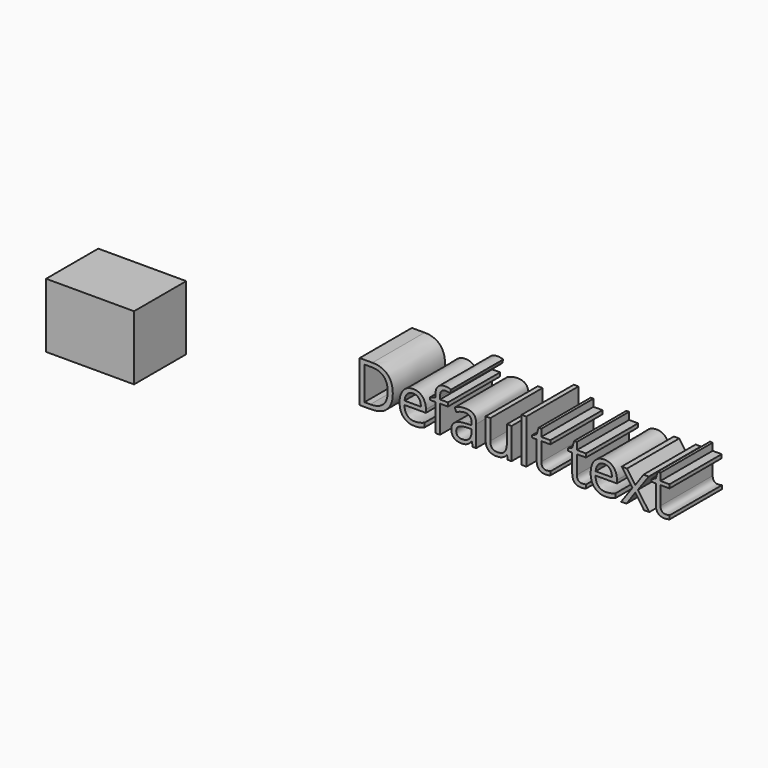
from build123d import *

# Parameters (mm, degrees)
F0_W         = 34.244004637
F0_H         = 25.0763148069
F1_DEPTH     = 25.4
F2_TEXT_SIZE = 22.6190003256
F3_DEPTH     = 25.4


# Not quite as in the source:
# - Text() gives the source's letters only with a copy of the font that has no kerning and outlines rounded to 1/6400 em; it was checked with that copy


with BuildPart() as f1:
    # F0 (on Front) → F1 (new body)
    with BuildSketch(Plane.XZ):
        with Locations((-53.9956521243, 29.0821269155)):
            Rectangle(F0_W, F0_H)
    extrude(amount=F1_DEPTH)


with BuildPart() as f3:
    # F2 (on face) → F3 (new body)
    with BuildSketch(Plane.XZ.offset(25.4)):
        with Locations((69.0735951066, 54.9350082874)):
            Text('Default text', F2_TEXT_SIZE, font='Open Sans', text_align=(TextAlign.LEFT, TextAlign.BOTTOM))
    extrude(amount=F3_DEPTH)


solid = Compound([f1.part, f3.part])
